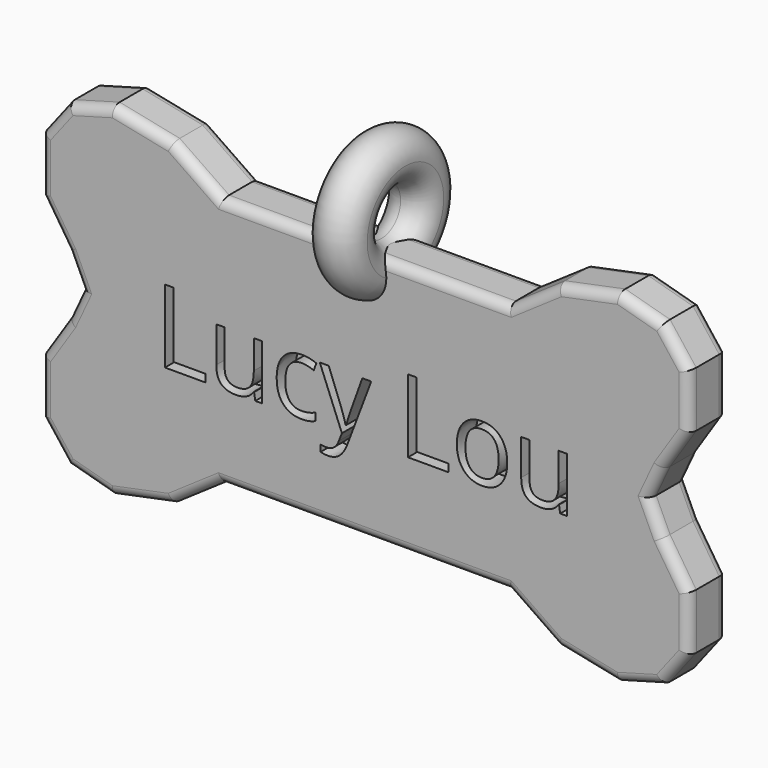
from build123d import *

# Parameters (mm, degrees)
F1_DEPTH     = 2.54
F2_R         = 0.508
F6_TEXT_SIZE = 5.4436916899
F7_DEPTH     = 1.27


# Not quite as in the source:
# - Text() gives the source's letters only with a copy of the font that has no kerning and outlines rounded to 1/6400 em; it was checked with that copy


with BuildPart() as f1:
    # F0 (on Front) → F1 (new body)
    with BuildSketch(Plane.XZ):
        Polygon((2.0103843274, 6.6693559441), (-5.6096156726, 6.6693559441), (-13.2296156726, 6.6693559441), (-15.8515510253, 8.4719367156), (-19.0470352022, 9.127420742), (-21.4231646474, 8.4719367156), (-22.8160668483, 6.6693559441), (-22.8160668483, 3.7196781265), (-21.4231646474, 1.5893559441), (-20.6857440637, 0), (-21.4231646474, -1.5893559441), (-22.8160668483, -3.7196781265), (-22.8160668483, -6.6693559441), (-21.4231646474, -8.4719367156), (-19.0470352022, -9.127420742), (-15.8515510253, -8.4719367156), (-13.2296156726, -6.6693559441), (-5.6096156726, -6.6693559441), (2.0103843274, -6.6693559441), (4.6323196802, -8.4719367156), (7.8278038571, -9.127420742), (10.2039333023, -8.4719367156), (11.5968355032, -6.6693559441), (11.5968355032, -3.7196781265), (10.2039333023, -1.5893559441), (9.4665127186, 0), (10.2039333023, 1.5893559441), (11.5968355032, 3.7196781265), (11.5968355032, 6.6693559441), (10.2039333023, 8.4719367156), (7.8278038571, 9.127420742), (4.6323196802, 8.4719367156), align=None)
    extrude(amount=F1_DEPTH)

    # F2
    f2_edges = [f1.edges().sort_by_distance(p)[0] for p in [
        (6.230062, -2.54, 8.799679),
        (3.321352, -2.54, 7.570646),
        (-5.609616, -2.54, 6.669356),
        (-14.540583, -2.54, 7.570646),
        (-17.449293, -2.54, 8.799679),
        (-20.2351, -2.54, 8.799679),
        (-22.119616, -2.54, 7.570646),
        (-22.816067, -2.54, 5.194517),
        (-22.119616, -2.54, 2.654517),
        (-21.054454, -2.54, 0.794678),
        (-21.054454, -2.54, -0.794678),
        (-22.119616, -2.54, -2.654517),
        (-22.816067, -2.54, -5.194517),
        (-22.119616, -2.54, -7.570646),
        (-20.2351, -2.54, -8.799679),
        (-17.449293, -2.54, -8.799679),
        (-14.540583, -2.54, -7.570646),
        (-5.609616, -2.54, -6.669356),
        (3.321352, -2.54, -7.570646),
        (6.230062, -2.54, -8.799679),
        (9.015869, -2.54, -8.799679),
        (10.900384, -2.54, -7.570646),
        (11.596836, -2.54, -5.194517),
        (10.900384, -2.54, -2.654517),
        (9.835223, -2.54, -0.794678),
        (9.835223, -2.54, 0.794678),
        (10.900384, -2.54, 2.654517),
        (11.596836, -2.54, 5.194517),
        (10.900384, -2.54, 7.570646),
        (9.015869, -2.54, 8.799679),
        (6.230062, 0, 8.799679),
        (3.321352, 0, 7.570646),
        (-5.609616, 0, 6.669356),
        (-14.540583, 0, 7.570646),
        (-17.449293, 0, 8.799679),
        (-20.2351, 0, 8.799679),
        (-22.119616, 0, 7.570646),
        (-22.816067, 0, 5.194517),
        (-22.119616, 0, 2.654517),
        (-21.054454, 0, 0.794678),
        (-21.054454, 0, -0.794678),
        (-22.119616, 0, -2.654517),
        (-22.816067, 0, -5.194517),
        (-22.119616, 0, -7.570646),
        (-20.2351, 0, -8.799679),
        (-17.449293, 0, -8.799679),
        (-14.540583, 0, -7.570646),
        (-5.609616, 0, -6.669356),
        (3.321352, 0, -7.570646),
        (6.230062, 0, -8.799679),
        (9.015869, 0, -8.799679),
        (10.900384, 0, -7.570646),
        (11.596836, 0, -5.194517),
        (10.900384, 0, -2.654517),
        (9.835223, 0, -0.794678),
        (9.835223, 0, 0.794678),
        (10.900384, 0, 2.654517),
        (11.596836, 0, 5.194517),
        (10.900384, 0, 7.570646),
        (9.015869, 0, 8.799679),
    ]]
    fillet(f2_edges, radius=F2_R)

    # F4 (on offset) → F5 (revolve)
    with BuildSketch(Plane.XZ.offset(1.27)):
        with BuildLine():
            ThreePointArc((-5.7404, 6.7623230782), (-6.6384256121, 4.5942974661), (-4.4704, 5.4923230782))
            ThreePointArc((-4.4704, 5.4923230782), (-4.8423743879, 6.3903486903), (-5.7404, 6.7623230782))
        make_face()
    revolve(axis=Axis((-2.6754314768, -1.27, 8.0323230782), (1, 0, 0)))

    # F6 (on face) → F7 (cut)
    with BuildSketch(Plane.XZ.offset(2.54)):
        with Locations((-16.7692750692, -2.1686488762)):
            Text('Lucy Lou', F6_TEXT_SIZE, font='Open Sans', text_align=(TextAlign.LEFT, TextAlign.BOTTOM))
    extrude(amount=-F7_DEPTH, mode=Mode.SUBTRACT)


solid = f1.part
